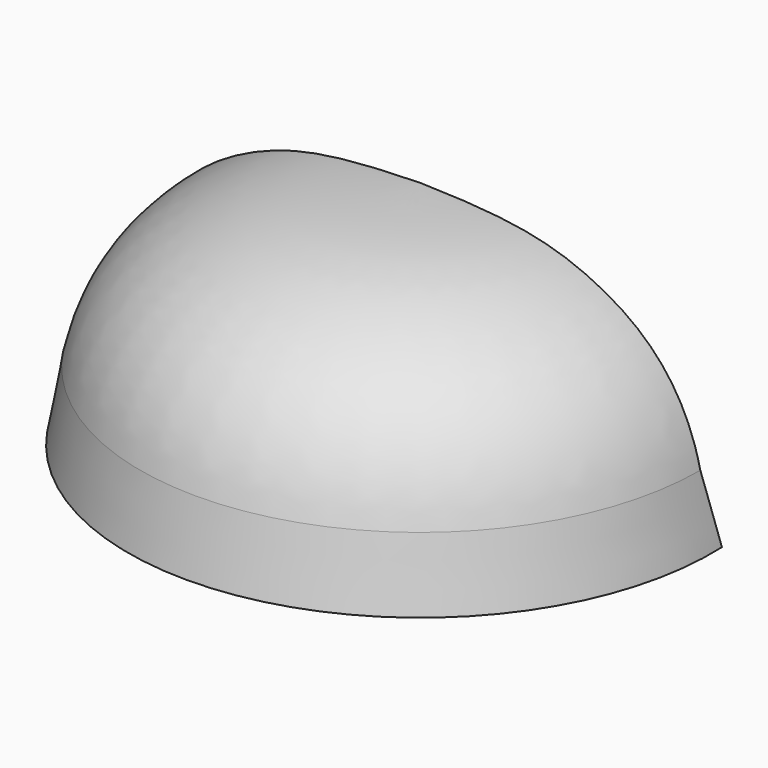
from build123d import *

# Parameters (mm, degrees)
F1_ANGLE_BACK          = 90
F1_ANGLE               = 180
F2_DEPTH               = 25
DRAFT_F2_DRAFTED_ANGLE = -10


# Not quite as in the source:
# - an extrude with a draft is written as a straight extrude whose walls are then drafted


with BuildPart() as f1:
    # F0 (on Right) → F1 (revolve)
    with BuildSketch(Plane.YZ, mode=Mode.PRIVATE) as f1_sk:
        with BuildLine():
            Line((0, 83.3354219794), (0, 142.2158185322))
            add(Edge.make_bspline(
                [(0, 142.2158185322), (-30.8364728954, 141.5517748026), (-61.8887228872, 136.7540358653), (-95.6590131206, 110.6618472068), (-101.8079742789, 83.3354219794)],
                knots=[0, 0, 0, 0, 0.5038552732, 1, 1, 1, 1], degree=3))
            Line((-101.8079742789, 83.3354219794), (0, 83.3354219794))
        make_face()
    revolve(f1_sk.sketch.rotate(Axis((0, 0, 112.7756202558), (0, 0, -1)), -F1_ANGLE_BACK), axis=Axis((0, 0, 112.7756202558), (0, 0, -1)), revolution_arc=F1_ANGLE)


with BuildPart() as f2_drafted:
    # F2 (new): a face of the model
    f2_faces = [f1.part.faces().sort_by_distance(p)[0] for p in [
        (0, -43.2086462738, 83.3354219794),
    ]]
    extrude(f2_faces, amount=F2_DEPTH)

    # draft_F2_drafted
    draft_f2_drafted_walls = [f2_drafted.faces().sort_by_distance(p)[0] for p in [
        (0, -101.8079742789, 66.6687553128),
        (0, 0, 66.6687553128),
    ]]
    draft(draft_f2_drafted_walls, neutral_plane=Plane(origin=(0, -43.2086462738, 83.3354219794), x_dir=(1, 0, 0), z_dir=(0, 0, -1)), angle=DRAFT_F2_DRAFTED_ANGLE)


with BuildPart() as f1_1:
    add(f1.part)

    # join_F2_drafted: union F2_drafted
    add(f2_drafted.part)


solid = f1_1.part
